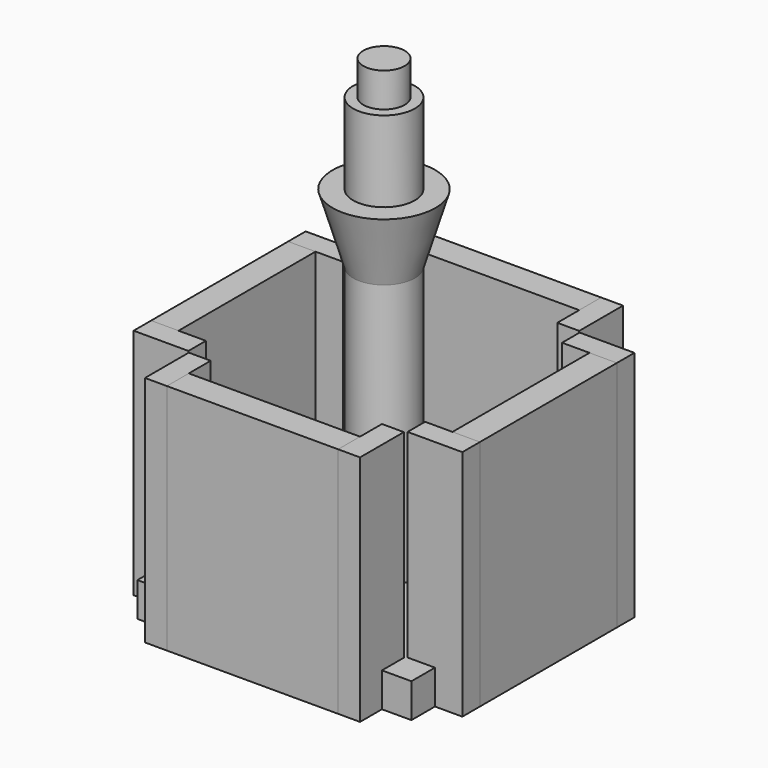
from build123d import *

# Parameters (mm, degrees)
F0_R              = 4.5
F1_DEPTH          = 70.43
F2_R              = 4.5
F2_R_2            = 3.025
F3_DEPTH          = 5
F4_W              = 40
F4_H              = 40
F4_R              = 4.5
F5_DEPTH          = 5
F6_W              = 25
F6_H              = 29
F6_H_2            = 5
F7_DEPTH          = 4
F7_COPIES_COUNT   = 4
F8_W              = 3.2
F8_H              = 29
F8_H_2            = 5
F9_DEPTH          = 4
F9_COPIES_COUNT   = 4
F9_2_COPIES_COUNT = 4
F10_R             = 3.175
F11_DEPTH         = 1.5
F12_W             = 9.8
F12_H             = 16.7
F13_DEPTH         = 5
F13_COPIES_COUNT  = 4
F18_R             = 4.5
F16_R             = 7.5


# Not quite as in the source:
# - a pattern or mirror of a feature is missing from the dataset's text; its kind, count and spacing are read off the source's solid


with BuildPart() as f1:
    # F0 (on Top) → F1 (new body)
    with BuildSketch(Plane.XY):
        Circle(F0_R)
    extrude(amount=F1_DEPTH)

    # F2 (on face) → F3 (cut)
    with BuildSketch(Plane.XY.offset(70.43)):
        Circle(F2_R)
        Circle(F2_R_2, mode=Mode.SUBTRACT)
    extrude(amount=-F3_DEPTH, mode=Mode.SUBTRACT)

    # F4 (on face) → F5 (join)
    with BuildSketch(Plane(origin=(0, 0, 0), x_dir=(1, 0, 0), z_dir=(0, 0, -1))):
        Rectangle(F4_W, F4_H)
        Circle(F4_R, mode=Mode.SUBTRACT)
    extrude(amount=-F5_DEPTH)

    # F6 (on face) → F7 (join)
    with BuildSketch(Plane(origin=(-20, 0, 0), x_dir=(0, -1, 0), z_dir=(-1, 0, 0))):
        with Locations((0, 19.5)):
            Rectangle(F6_W, F6_H)
        with Locations((0, 2.5)):
            Rectangle(F6_W, F6_H_2)
    f7 = extrude(amount=F7_DEPTH)

    # F7_copies: F7 ×4 about axis
    f7_copies_axis = Axis((0, 0, 0), (0, 0, 1))
    for i in range(1, F7_COPIES_COUNT):
        add(f7.rotate(f7_copies_axis, i * 360 / F7_COPIES_COUNT))

    # F10 (on face) → F11 (cut)
    with BuildSketch(Plane(origin=(0, 0, 0), x_dir=(1, 0, 0), z_dir=(0, 0, -1))):
        Circle(F10_R)
    extrude(amount=-F11_DEPTH, mode=Mode.SUBTRACT)

    # F12 (on face) → F13 (cut)
    with BuildSketch(Plane.XY.offset(5)):
        with Locations((15.1, 0)):
            Rectangle(F12_W, F12_H)
    f13 = extrude(amount=-F13_DEPTH, mode=Mode.SUBTRACT)

    # F13_copies: F13 ×4 about axis
    f13_copies_axis = Axis((0, 0, 0), (0, 0, 1))
    for i in range(1, F13_COPIES_COUNT):
        add(f13.rotate(f13_copies_axis, i * 360 / F13_COPIES_COUNT), mode=Mode.SUBTRACT)

    # F18 (on offset) → F19 section 0
    with BuildSketch(Plane.XY.offset(43.63)):
        Circle(F18_R)
    # F16 (on offset) → F19 section 1
    with BuildSketch(Plane.XY.offset(53.63)):
        Circle(F16_R)
    loft()


with BuildPart() as f9:
    # F8 (on face) → F9 (new body, symmetric)
    with BuildSketch(Plane(origin=(-20, 0, 0), x_dir=(0, -1, 0), z_dir=(-1, 0, 0))):
        with Locations((-14.1, 19.5)):
            Rectangle(F8_W, F8_H)
        with Locations((-14.1, 2.5)):
            Rectangle(F8_W, F8_H_2)
    extrude(amount=F9_DEPTH, both=True)


with BuildPart() as f9b:
    # F8 (on face) → F9, piece 2 (new body, symmetric)
    with BuildSketch(Plane(origin=(-20, 0, 0), x_dir=(0, -1, 0), z_dir=(-1, 0, 0))):
        with Locations((14.1, 19.5)):
            Rectangle(F8_W, F8_H)
        with Locations((14.1, 2.5)):
            Rectangle(F8_W, F8_H_2)
    extrude(amount=F9_DEPTH, both=True)


with BuildPart() as f9_copies_1:
    # F9_copies: instance of F9
    add(f9.part.rotate(Axis((0, 0, 0), (0, 0, 1)), 1 * 360 / F9_COPIES_COUNT))


with BuildPart() as f9_copies_2:
    # F9_copies: instance of F9
    add(f9.part.rotate(Axis((0, 0, 0), (0, 0, 1)), 2 * 360 / F9_COPIES_COUNT))


with BuildPart() as f9_copies_3:
    # F9_copies: instance of F9
    add(f9.part.rotate(Axis((0, 0, 0), (0, 0, 1)), 3 * 360 / F9_COPIES_COUNT))


with BuildPart() as f9_2_copies_1:
    # F9_2_copies: instance of F9b
    add(f9b.part.rotate(Axis((0, 0, 0), (0, 0, 1)), 1 * 360 / F9_2_COPIES_COUNT))


with BuildPart() as f9_2_copies_2:
    # F9_2_copies: instance of F9b
    add(f9b.part.rotate(Axis((0, 0, 0), (0, 0, 1)), 2 * 360 / F9_2_COPIES_COUNT))


with BuildPart() as f9_2_copies_3:
    # F9_2_copies: instance of F9b
    add(f9b.part.rotate(Axis((0, 0, 0), (0, 0, 1)), 3 * 360 / F9_2_COPIES_COUNT))


solid = Compound([f1.part, f9.part, f9b.part, f9_copies_1.part, f9_copies_2.part, f9_copies_3.part, f9_2_copies_1.part, f9_2_copies_2.part, f9_2_copies_3.part])
